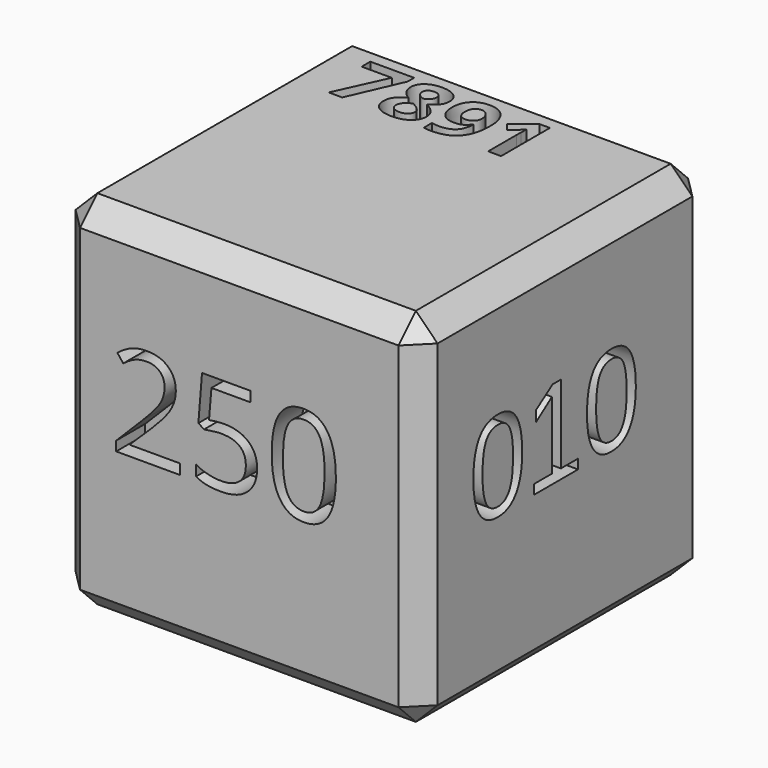
from build123d import *

# Parameters (mm, degrees)
F0_W          = 50
F0_H          = 50
F1_DEPTH      = 50
F2_SIZE       = 3
F3_TEXT_SIZE  = 11.818854785
F4_DEPTH      = 5
F5_TEXT_SIZE  = 35.3535365624
F6_DEPTH      = 5
F7_TEXT_SIZE  = 16.3133282007
F8_DEPTH      = 5
F9_TEXT_SIZE  = 17.6411303174
F11_DEPTH     = 5
F10_TEXT_SIZE = 18.7779518051
F12_DEPTH     = 5
F13_TEXT_SIZE = 19.7147743569
F14_DEPTH     = 5


# Not quite as in the source:
# - Text() gives the source's letters only with a copy of the font that has no kerning and outlines rounded to 1/6400 em; it was checked with that copy


with BuildPart() as f1:
    # F0 (on Top) → F1 (new body)
    with BuildSketch(Plane.XY):
        with Locations((-7.3686908349, -0.9616399184)):
            Rectangle(F0_W, F0_H)
    extrude(amount=F1_DEPTH)

    # F2
    f2_edges = [f1.edges().sort_by_distance(p)[0] for p in [
        (17.631309, -0.96164, 50),
        (-7.368691, -25.96164, 50),
        (-32.368691, -0.96164, 50),
        (-7.368691, 24.03836, 50),
        (-7.368691, -25.96164, 0),
        (-32.368691, -0.96164, 0),
        (-7.368691, 24.03836, 0),
        (17.631309, -0.96164, 0),
        (17.631309, 24.03836, 25),
        (-32.368691, 24.03836, 25),
        (-32.368691, -25.96164, 25),
        (17.631309, -25.96164, 25),
    ]]
    chamfer(f2_edges, length=F2_SIZE)

    # F3 (on face) → F4 (cut)
    with BuildSketch(Plane.XY.offset(50)):
        with Locations((-25.8869853713, 11.0018644561)):
            Text('7891', F3_TEXT_SIZE, font='Open Sans', font_style=FontStyle.BOLD, text_align=(TextAlign.LEFT, TextAlign.BOTTOM))
    extrude(amount=-F4_DEPTH, mode=Mode.SUBTRACT)

    # F5 (on face) → F6 (cut)
    with BuildSketch(Plane(origin=(0, 0, 0), x_dir=(1, 0, 0), z_dir=(0, 0, -1))):
        with Locations((-17.1590913087, -11.5909092128)):
            Text('2', F5_TEXT_SIZE, font='Open Sans', text_align=(TextAlign.LEFT, TextAlign.BOTTOM))
    extrude(amount=-F6_DEPTH, mode=Mode.SUBTRACT)

    # F7 (on face) → F8 (cut)
    with BuildSketch(Plane(origin=(0, 24.0383600816, 0), x_dir=(-1, 0, 0), z_dir=(0, 1, 0))):
        with Locations((-11.110201478, 20.7604598254)):
            Text('2017', F7_TEXT_SIZE, font='Open Sans', text_align=(TextAlign.LEFT, TextAlign.BOTTOM))
    extrude(amount=-F8_DEPTH, mode=Mode.SUBTRACT)

    # F9 (on face) → F11 (cut)
    with BuildSketch(Plane.YZ.offset(17.6313091651)):
        with Locations((-17.4647178501, 21.8245964497)):
            Text('010', F9_TEXT_SIZE, font='Arimo', text_align=(TextAlign.LEFT, TextAlign.BOTTOM))
    extrude(amount=-F11_DEPTH, mode=Mode.SUBTRACT)

    # F10 (on face) → F12 (cut)
    with BuildSketch(Plane.XZ.offset(25.9616399184)):
        with Locations((-25.288971141, 21.4350447059)):
            Text('250', F10_TEXT_SIZE, font='Open Sans', text_align=(TextAlign.LEFT, TextAlign.BOTTOM))
    extrude(amount=-F12_DEPTH, mode=Mode.SUBTRACT)

    # F13 (on face) → F14 (cut)
    with BuildSketch(Plane(origin=(-32.3686908349, 0, 0), x_dir=(0, -1, 0), z_dir=(-1, 0, 0))):
        with Locations((-13.6096561328, 21.2985761464)):
            Text('011', F13_TEXT_SIZE, font='Open Sans', text_align=(TextAlign.LEFT, TextAlign.BOTTOM))
    extrude(amount=-F14_DEPTH, mode=Mode.SUBTRACT)


solid = f1.part
